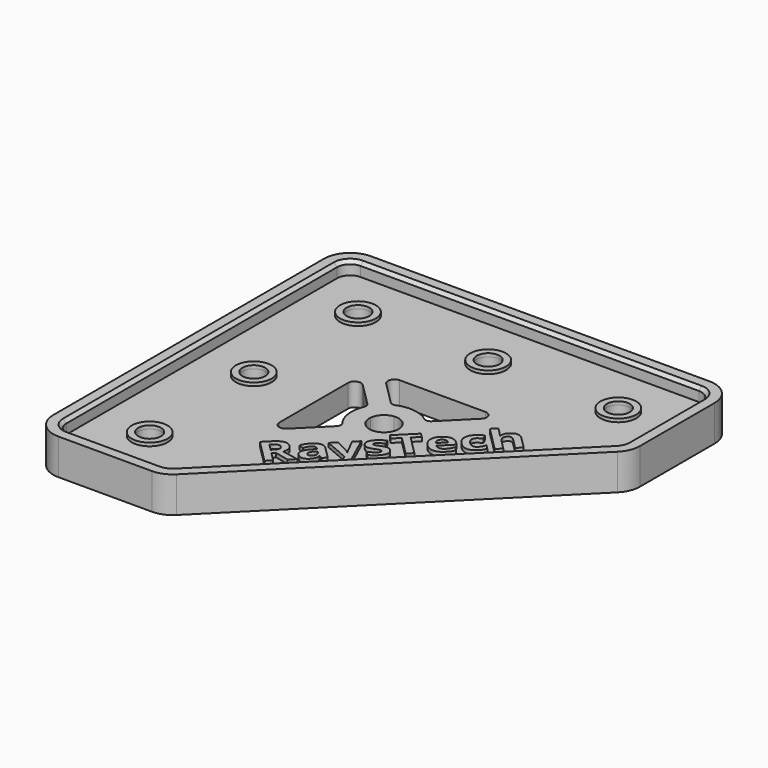
from build123d import *

# Parameters (mm, degrees)
F1_DEPTH     = 5.5
F2_R         = 4
F3_T         = -2
F4_DEPTH     = 1.5
F5_R         = 1.75
F6_DEPTH     = 25
F7_R         = 1
F8_R         = 0.8
F9_TEXT_SIZE = 6.9444444444
F10_DEPTH    = 0.6
F11_SIZE     = 0.5
F12_R        = 2.75
F12_R_2      = 1.75
F13_DEPTH    = 0.5


# Not quite as in the source:
# - Text() gives the source's letters only with a copy of the font that has no kerning and outlines rounded to 1/6400 em; it was checked with that copy


with BuildPart() as f1:
    # F0 (on Top) → F1 (new body)
    with BuildSketch(Plane.XY):
        Polygon((14.2679563351, 7.8787696362), (-45.7320436649, 7.8787696362), (-45.7320436649, -52.1212303638), (-25.7320436649, -52.1212303638), (14.2679563351, -12.1212303638), align=None)
    extrude(amount=F1_DEPTH)

    # F2
    f2_edges = [f1.edges().sort_by_distance(p)[0] for p in [
        (14.267956, -12.12123, 2.75),
        (14.267956, 7.87877, 2.75),
        (-25.732044, -52.12123, 2.75),
        (-45.732044, -52.12123, 2.75),
        (-45.732044, 7.87877, 2.75),
    ]]
    fillet(f2_edges, radius=F2_R)

    # F3
    f3_openings = [f1.faces().sort_by_distance(p)[0] for p in [
        (-20.479304, -17.37397, 5.5),
    ]]
    offset(amount=F3_T, openings=f3_openings)

    # F4 (add): a face of the model
    f4_faces = [f1.faces().sort_by_distance(p)[0] for p in [
        (-20.492964184, -17.3603098448, 2),
    ]]
    extrude(f4_faces, amount=F4_DEPTH)

    # F5 (on face) → F6 (cut)
    with BuildSketch(Plane.XY.offset(3.5)):
        with Locations((-35.7320436649, -2.1212303638)):
            Circle(F5_R)
        with Locations((-35.7320436649, -22.1212303638)):
            Circle(F5_R)
        with Locations((-35.7320436649, -42.1212303638)):
            Circle(F5_R)
        with Locations((-15.7320436649, -2.1212303638)):
            Circle(F5_R)
        with Locations((4.2679563351, -2.1212303638)):
            Circle(F5_R)
        with BuildLine():
            Line((-20.123112756, -19.7301612727), (-25.7320436649, -14.1212303638))
            Line((-25.7320436649, -14.1212303638), (-25.7320436649, -32.1214221648))
            Line((-25.7320436649, -32.1214221648), (-19.2674816704, -25.6568601702))
            ThreePointArc((-19.2674816704, -25.6568601702), (-20.6806424214, -22.8357639395), (-20.123112756, -19.7301612727))
        make_face()
        with BuildLine():
            Line((-23.7320436649, -12.1212303638), (-18.123112756, -17.7301612727))
            ThreePointArc((-18.123112756, -17.7301612727), (-15.0175100893, -17.1726316073), (-12.1964138585, -18.5857923584))
            Line((-12.1964138585, -18.5857923584), (-5.731851864, -12.1212303638))
            Line((-5.731851864, -12.1212303638), (-23.7320436649, -12.1212303638))
        make_face()
        with BuildLine():
            ThreePointArc((-15.9693846315, -19.8838893972), (-17.3229380221, -20.5303360066), (-17.9693846315, -21.8838893972))
            Line((-17.9693846315, -21.8838893972), (-16.7319477644, -23.1213262643))
            Line((-16.7319477644, -23.1213262643), (-17.3229380221, -23.712316522))
            ThreePointArc((-17.3229380221, -23.712316522), (-14.8709100416, -24.2000552125), (-13.4819477644, -22.1213262643))
            ThreePointArc((-13.4819477644, -22.1213262643), (-13.6532188163, -21.2602885415), (-14.1409575068, -20.5303360066))
            Line((-14.1409575068, -20.5303360066), (-14.7319477644, -21.1213262643))
            Line((-14.7319477644, -21.1213262643), (-15.9693846315, -19.8838893972))
        make_face()
        with BuildLine():
            ThreePointArc((-14.1409575068, -20.5303360066), (-14.9819477644, -20.0000059207), (-15.9693846315, -19.8838893972))
            Line((-15.9693846315, -19.8838893972), (-14.7319477644, -21.1213262643))
            Line((-14.7319477644, -21.1213262643), (-14.1409575068, -20.5303360066))
        make_face()
        with BuildLine():
            Line((-16.7319477644, -23.1213262643), (-17.9693846315, -21.8838893972))
            ThreePointArc((-17.9693846315, -21.8838893972), (-17.853268108, -22.8713262643), (-17.3229380221, -23.712316522))
            Line((-17.3229380221, -23.712316522), (-16.7319477644, -23.1213262643))
        make_face()
    extrude(amount=-F6_DEPTH, mode=Mode.SUBTRACT)

    # F7
    f7_edges = [f1.edges().sort_by_distance(p)[0] for p in [
        (-23.732044, -12.12123, 1.75),
        (-25.732044, -14.12123, 1.75),
        (-5.731852, -12.12123, 1.75),
        (-25.732044, -32.121422, 1.75),
    ]]
    fillet(f7_edges, radius=F7_R)

    # F8
    f8_edges = [f1.edges().sort_by_distance(p)[0] for p in [
        (-12.196414, -18.585792, 1.75),
        (-18.123113, -17.730161, 1.75),
        (-19.267482, -25.65686, 1.75),
        (-20.123113, -19.730161, 1.75),
    ]]
    fillet(f8_edges, radius=F8_R)

    # F9 (on face) → F10 (join)
    with BuildSketch(Plane.XY.offset(3.5)):
        with Locations(Location((-20.6296326372, -39.9477515243), (0, 0, 45))):
            Text('RaysTech', F9_TEXT_SIZE, font='Open Sans', font_style=FontStyle.BOLD, text_align=(TextAlign.LEFT, TextAlign.BOTTOM))
    extrude(amount=F10_DEPTH)

    # F11
    f11_edges = [f1.edges().sort_by_distance(p)[0] for p in [
        (-15.732044, 5.87877, 5.5),
    ]]
    chamfer(f11_edges, length=F11_SIZE)

    # F12 (on face) → F13 (join)
    with BuildSketch(Plane.XY.offset(3.5)):
        with Locations((-35.7320436649, -2.1212303638)):
            Circle(F12_R)
        with Locations((-35.7320436649, -2.1212303638)):
            Circle(F12_R_2, mode=Mode.SUBTRACT)
        with Locations((-35.7320436649, -22.1212303638)):
            Circle(F12_R)
        with Locations((-35.7320436649, -22.1212303638)):
            Circle(F12_R_2, mode=Mode.SUBTRACT)
        with Locations((-35.7320436649, -42.1212303638)):
            Circle(F12_R)
        with Locations((-35.7320436649, -42.1212303638)):
            Circle(F12_R_2, mode=Mode.SUBTRACT)
        with Locations((-15.7320436649, -2.1212303638)):
            Circle(F12_R)
        with Locations((-15.7320436649, -2.1212303638)):
            Circle(F12_R_2, mode=Mode.SUBTRACT)
        with Locations((4.2679563351, -2.1212303638)):
            Circle(F12_R)
        with Locations((4.2679563351, -2.1212303638)):
            Circle(F12_R_2, mode=Mode.SUBTRACT)
    extrude(amount=F13_DEPTH)


solid = f1.part
